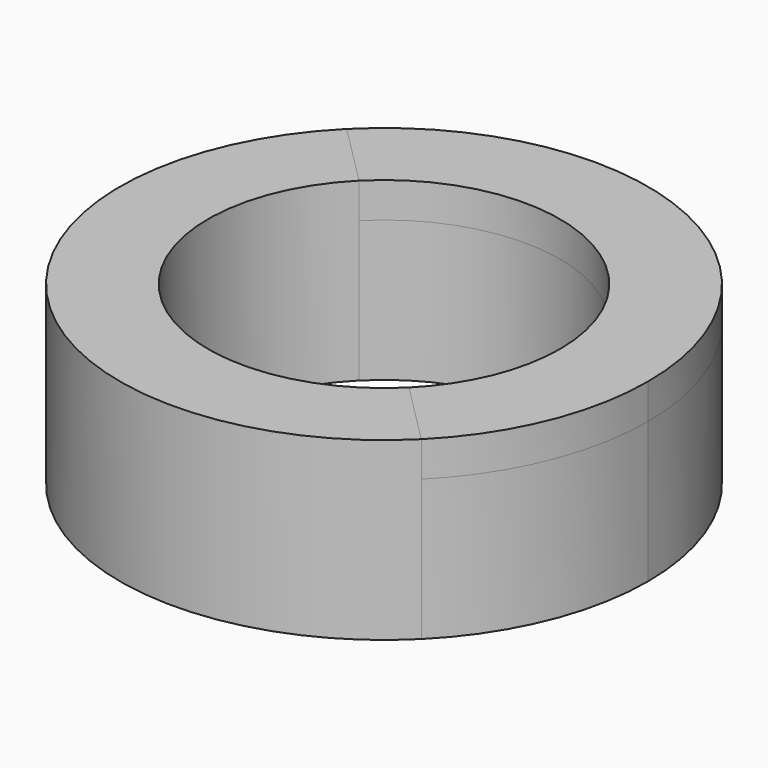
from build123d import *
from build123d import SkipClean  # not in build123d's __all__

# Parameters (mm, degrees)
F1_DEPTH = 25.4
F2_DEPTH = 31.75
F3_DEPTH = 6.35


with BuildPart() as f1:
    # F0 (on Top) → F1 (new body)
    with BuildSketch(Plane.XY):
        with BuildLine():
            ThreePointArc((33.675960454, -33.675960454), (43.9997627359, -18.2252984664), (47.625, 0))
            ThreePointArc((47.625, 0), (18.2252984664, 43.9997627359), (-33.675960454, 33.675960454))
            Line((-33.675960454, 33.675960454), (-22.4506403027, 22.4506403027))
            ThreePointArc((-22.4506403027, 22.4506403027), (12.1501989776, 29.3331751572), (31.75, 0))
            ThreePointArc((31.75, 0), (29.3331751572, -12.1501989776), (22.4506403027, -22.4506403027))
            Line((22.4506403027, -22.4506403027), (33.675960454, -33.675960454))
        make_face()
    extrude(amount=F1_DEPTH)


with BuildPart() as f2:
    # F0 (on Top) → F2 (new body)
    with BuildSketch(Plane.XY):
        with BuildLine():
            Line((-22.4506403027, 22.4506403027), (-33.675960454, 33.675960454))
            ThreePointArc((-33.675960454, 33.675960454), (-33.675960454, -33.675960454), (33.675960454, -33.675960454))
            Line((33.675960454, -33.675960454), (22.4506403027, -22.4506403027))
            ThreePointArc((22.4506403027, -22.4506403027), (-22.4506403027, -22.4506403027), (-22.4506403027, 22.4506403027))
        make_face()
    extrude(amount=F2_DEPTH)

    # F3 (add): a face of the model
    f3_faces = [f1.part.faces().sort_by_distance(p)[0] for p in [
        (32.8629508495, 32.8629508495, 25.4),
    ]]
    with SkipClean():  # cleaning this boolean's faces spoils the solid; the shape is the same uncleaned
        extrude(f3_faces, amount=F3_DEPTH)


solid = Compound([f1.part, f2.part])
